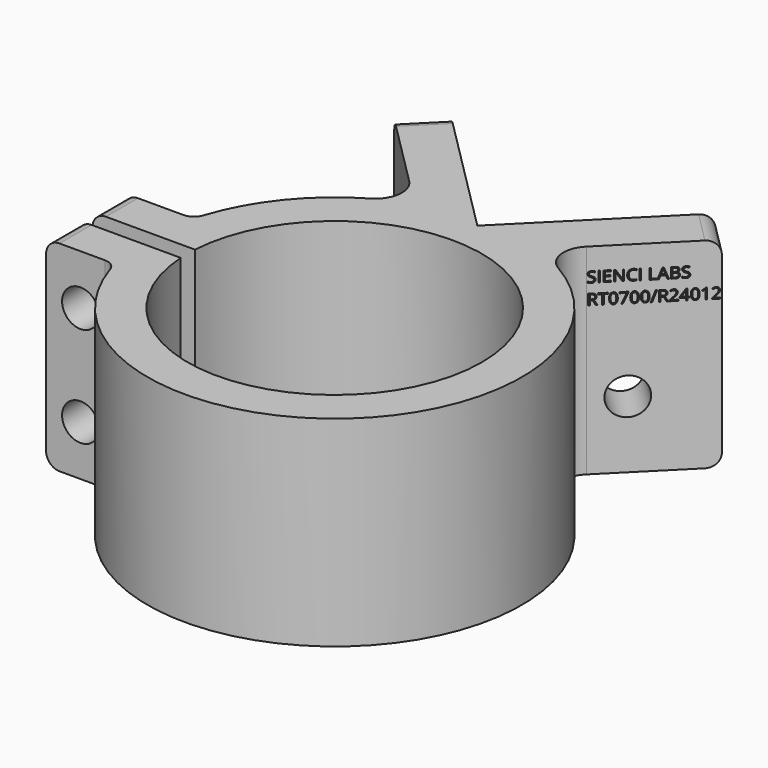
from build123d import *

# Parameters (mm, degrees)
F1_DEPTH      = 45
F2_R          = 4.125
F3_DEPTH      = 10
F4_R          = 4.125
F5_DEPTH      = 10
F6_R          = 4.125
F7_DEPTH      = 22
F8_R          = 3
F10_DEPTH     = 3
F11_R         = 6
F12_TEXT_SIZE = 3.2656050492
F13_DEPTH     = 0.5


# Not quite as in the source:
# - Text() gives the source's letters only with a copy of the font that has no kerning and outlines rounded to 1/6400 em; it was checked with that copy


with BuildPart() as f1:
    # F0 (on Top) → F1 (new body)
    with BuildSketch(Plane.XY):
        with BuildLine():
            Line((29.6984848098, 29.6984848098), (0, 0))
            Line((0, 0), (-29.6984848098, 29.6984848098))
            Line((-29.6984848098, 29.6984848098), (-36.7695526217, 22.627416998))
            Line((-36.7695526217, 22.627416998), (-13.8076104544, -0.3345251694))
            ThreePointArc((-13.8076104544, -0.3345251694), (-30.7193471679, -11.3587411314), (-40.533936399, -29))
            ThreePointArc((-40.533936399, -29), (-41.4879141791, -33.4614239264), (-41.9523539268, -38))
            Line((-41.9523539268, -38), (-32.939338184, -38))
            ThreePointArc((-32.939338184, -38), (33, -40), (-32.939338184, -42))
            Line((-32.939338184, -42), (-41.9523539268, -42))
            ThreePointArc((-41.9523539268, -42), (-41.4879141791, -46.5385760736), (-40.533936399, -51))
            ThreePointArc((-40.533936399, -51), (28.6412588686, -70.7193471679), (13.8076104544, -0.3345251694))
            Line((13.8076104544, -0.3345251694), (36.7695526217, 22.627416998))
            Line((36.7695526217, 22.627416998), (29.6984848098, 29.6984848098))
        make_face()
        with BuildLine():
            ThreePointArc((-41.9523539268, -38), (-41.4879141791, -33.4614239264), (-40.533936399, -29))
            Line((-40.533936399, -29), (-55.9523539268, -29))
            Line((-55.9523539268, -29), (-55.9523539268, -38))
            Line((-55.9523539268, -38), (-41.9523539268, -38))
        make_face()
        with BuildLine():
            Line((-55.9523539268, -51), (-40.533936399, -51))
            ThreePointArc((-40.533936399, -51), (-41.4879141791, -46.5385760736), (-41.9523539268, -42))
            Line((-41.9523539268, -42), (-55.9523539268, -42))
            Line((-55.9523539268, -42), (-55.9523539268, -51))
        make_face()
    extrude(amount=F1_DEPTH)

    # F2 (on face) → F3 (cut, through all)
    with BuildSketch(Plane(origin=(0, 0, 0), x_dir=(-0.7071067812, -0.7071067812, 0), z_dir=(-0.7071067812, 0.7071067812, 0))):
        with Locations((-25.4, 15)):
            Circle(F2_R)
    extrude(amount=-F3_DEPTH, mode=Mode.SUBTRACT)

    # F4 (on face) → F5 (cut, through all)
    with BuildSketch(Plane(origin=(0, 0, 0), x_dir=(-0.7071067812, 0.7071067812, 0), z_dir=(0.7071067812, 0.7071067812, 0))):
        with Locations((25.4, 15)):
            Circle(F4_R)
    extrude(amount=-F5_DEPTH, mode=Mode.SUBTRACT)

    # F6 (on face) → F7 (cut, through all)
    with BuildSketch(Plane.XZ.offset(51)):
        with Locations((-48.2431451629, 33.75)):
            Circle(F6_R)
        with Locations((-48.2431451629, 11.25)):
            Circle(F6_R)
    extrude(amount=-F7_DEPTH, mode=Mode.SUBTRACT)

    # F8
    f8_edges = [f1.edges().sort_by_distance(p)[0] for p in [
        (-55.952354, -33.5, 45),
        (-55.952354, -46.5, 45),
        (-55.952354, -46.5, 0),
        (-55.952354, -33.5, 0),
        (-33.234019, 26.162951, 45),
        (33.234019, 26.162951, 45),
        (33.234019, 26.162951, 0),
        (-33.234019, 26.162951, 0),
        (-40.533936, -29, 22.5),
        (-40.533936, -51, 22.5),
    ]]
    fillet(f8_edges, radius=F8_R)

    # F9 (on face) → F10 (cut)
    with BuildSketch(Plane(origin=(0, -29, 0), x_dir=(-1, 0, 0), z_dir=(0, 1, 0))):
        Polygon((55.1681451629, 37.7481506141), (48.2431451629, 41.7463012283), (41.3181451629, 37.7481506141), (41.3181451629, 29.7518493859), (48.2431451629, 25.7536987717), (55.1681451629, 29.7518493859), align=None)
        Polygon((55.1681451629, 7.2518493859), (55.1681451629, 15.2481506141), (48.2431451629, 19.2463012283), (41.3181451629, 15.2481506141), (41.3181451629, 7.2518493859), (48.2431451629, 3.2536987717), align=None)
    extrude(amount=-F10_DEPTH, mode=Mode.SUBTRACT)

    # F11
    f11_edges = [f1.edges().sort_by_distance(p)[0] for p in [
        (-13.80761, -0.334525, 22.5),
        (13.80761, -0.334525, 22.5),
    ]]
    fillet(f11_edges, radius=F11_R)

    # F12 (on face) → F13 (cut)
    with BuildSketch(Plane(origin=(7.0710678119, -7.0710678119, 0), x_dir=(0.7071067812, 0.7071067812, 0), z_dir=(0.7071067812, -0.7071067812, 0))):
        with Locations((18.1172015731, 37.7863595759)):
            Text('SIENCI LABS', F12_TEXT_SIZE, font='Open Sans', text_align=(TextAlign.LEFT, TextAlign.BOTTOM))
        with Locations((18.1172015731, 33.3451367091)):
            Text('RT0700/R24012', F12_TEXT_SIZE, font='Open Sans', text_align=(TextAlign.LEFT, TextAlign.BOTTOM))
    extrude(amount=-F13_DEPTH, mode=Mode.SUBTRACT)


solid = f1.part
